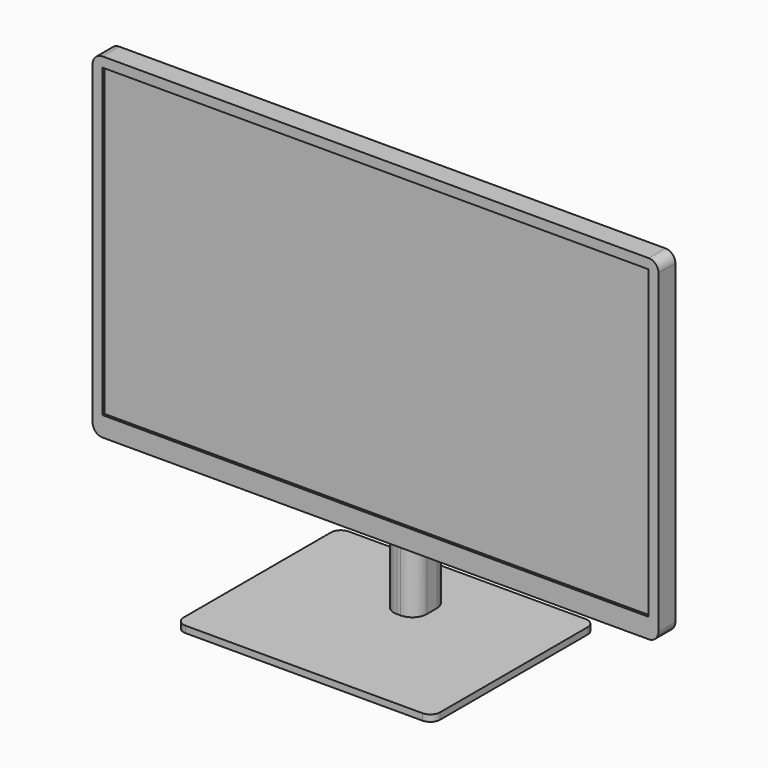
from build123d import *

# Parameters (mm, degrees)
F1_DEPTH = 6.35
F3_DEPTH = 114.3
F5_DEPTH = 101.6
F7_DEPTH = 20.32
F8_W     = 527.05
F8_H     = 295.275
F9_DEPTH = 2.54


with BuildPart() as f1:
    # F0 (on Top) → F1 (new body)
    with BuildSketch(Plane.XY):
        with BuildLine():
            Line((-114.3, -98.425), (114.3, -98.425))
            ThreePointArc((114.3, -98.425), (121.0351920908, -95.6351920908), (123.825, -88.9))
            Line((123.825, -88.9), (123.825, 88.9))
            ThreePointArc((123.825, 88.9), (121.0351920908, 95.6351920908), (114.3, 98.425))
            Line((114.3, 98.425), (-114.3, 98.425))
            ThreePointArc((-114.3, 98.425), (-121.0351920908, 95.6351920908), (-123.825, 88.9))
            Line((-123.825, 88.9), (-123.825, -88.9))
            ThreePointArc((-123.825, -88.9), (-121.0351920908, -95.6351920908), (-114.3, -98.425))
        make_face()
    extrude(amount=F1_DEPTH)

    # F2 (on face) → F3 (join)
    with BuildSketch(Plane.XY.offset(6.35)):
        with BuildLine():
            Line((-1.905, 15.875), (1.905, 15.875))
            ThreePointArc((1.905, 15.875), (11.7832817332, 19.9667182668), (15.875, 29.845))
            Line((15.875, 29.845), (15.875, 42.037))
            ThreePointArc((15.875, 42.037), (11.7832817332, 51.9152817332), (1.905, 56.007))
            Line((1.905, 56.007), (-1.905, 56.007))
            ThreePointArc((-1.905, 56.007), (-11.7832817332, 51.9152817332), (-15.875, 42.037))
            Line((-15.875, 42.037), (-15.875, 29.845))
            ThreePointArc((-15.875, 29.845), (-11.7832817332, 19.9667182668), (-1.905, 15.875))
        make_face()
    extrude(amount=F3_DEPTH)

    # F4 (on face) → F5 (join)
    with BuildSketch(Plane.XY.offset(120.65)):
        with BuildLine():
            ThreePointArc((-15.875, 42.037), (-13.9930859093, 49.0397908043), (-8.8543730782, 54.1558742802))
            Line((-8.8543730782, 54.1558742802), (-88.9, 8.255))
            Line((-88.9, 8.255), (88.9, 8.255))
            Line((88.9, 8.255), (8.8543730782, 54.1558742802))
            ThreePointArc((8.8543730782, 54.1558742802), (13.9930859093, 49.0397908043), (15.875, 42.037))
            Line((15.875, 42.037), (15.875, 29.845))
            ThreePointArc((15.875, 29.845), (11.7832817332, 19.9667182668), (1.905, 15.875))
            Line((1.905, 15.875), (-1.905, 15.875))
            ThreePointArc((-1.905, 15.875), (-11.7832817332, 19.9667182668), (-15.875, 29.845))
            Line((-15.875, 29.845), (-15.875, 42.037))
        make_face()
        with BuildLine():
            ThreePointArc((-1.905, 56.007), (-5.5008466531, 55.536288383), (-8.8543730782, 54.1558742802))
            ThreePointArc((-8.8543730782, 54.1558742802), (-13.9930859093, 49.0397908043), (-15.875, 42.037))
            Line((-15.875, 42.037), (-15.875, 29.845))
            ThreePointArc((-15.875, 29.845), (-11.7832817332, 19.9667182668), (-1.905, 15.875))
            Line((-1.905, 15.875), (1.905, 15.875))
            ThreePointArc((1.905, 15.875), (11.7832817332, 19.9667182668), (15.875, 29.845))
            Line((15.875, 29.845), (15.875, 42.037))
            ThreePointArc((15.875, 42.037), (13.9930859093, 49.0397908043), (8.8543730782, 54.1558742802))
            ThreePointArc((8.8543730782, 54.1558742802), (5.5008466531, 55.536288383), (1.905, 56.007))
            Line((1.905, 56.007), (-1.905, 56.007))
        make_face()
    extrude(amount=F5_DEPTH)

    # F6 (on face) → F7 (join)
    with BuildSketch(Plane.XZ.offset(-8.255)):
        with BuildLine():
            Line((263.525, 406.4), (-263.525, 406.4))
            ThreePointArc((-263.525, 406.4), (-270.2601920908, 403.6101920908), (-273.05, 396.875))
            Line((-273.05, 396.875), (-273.05, 92.075))
            ThreePointArc((-273.05, 92.075), (-270.2601920908, 85.3398079092), (-263.525, 82.55))
            Line((-263.525, 82.55), (263.525, 82.55))
            ThreePointArc((263.525, 82.55), (270.2601920908, 85.3398079092), (273.05, 92.075))
            Line((273.05, 92.075), (273.05, 396.875))
            ThreePointArc((273.05, 396.875), (270.2601920908, 403.6101920908), (263.525, 406.4))
        make_face()
    extrude(amount=F7_DEPTH)

    # F8 (on face) → F9 (cut)
    with BuildSketch(Plane.XZ.offset(12.065)):
        with Locations((0, 249.2375)):
            Rectangle(F8_W, F8_H)
    extrude(amount=-F9_DEPTH, mode=Mode.SUBTRACT)


solid = f1.part
